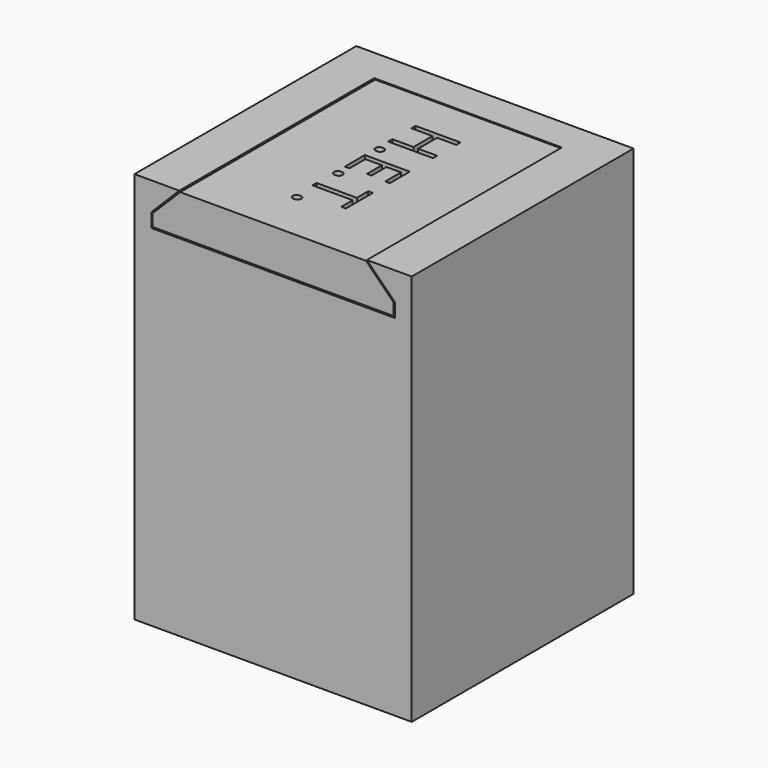
from build123d import *

# Parameters (mm, degrees)
F1_DEPTH      = 25
F2_W          = 19.8
F2_H          = 19.8
F3_DEPTH      = 1
F5_DEPTH      = 2
F7_DEPTH      = 1
F8_DEPTH      = 19.8
F10_DEPTH     = 2.4
F11_DEPTH     = 2
F13_DEPTH     = 17.4
F14_TEXT_SIZE = 4.4975727279
F15_DEPTH     = 3


# Not quite as in the source:
# - Text() gives the source's letters only with a copy of the font that has no kerning and outlines rounded to 1/6400 em; it was checked with that copy


with BuildPart() as f1:
    # F0 (on Top) → F1 (new body)
    with BuildSketch(Plane.XY):
        Polygon((0, -7.5), (-7.5, -7.5), (-7.5, 0), (-7.5, 7.5), (-7.5, 9.9), (-9.9, 9.9), (-9.9, -9.9), (9.9, -9.9), (9.9, -7.5), (7.5, -7.5), align=None)
        Polygon((7.5, 7.5), (7.5, -7.5), (9.9, -7.5), (9.9, 9.9), (-7.5, 9.9), (-7.5, 7.5), align=None)
    extrude(amount=F1_DEPTH)

    # F2 (on face) → F3 (join)
    with BuildSketch(Plane(origin=(0, 0, 0), x_dir=(1, 0, 0), z_dir=(0, 0, -1))):
        Rectangle(F2_W, F2_H)
    extrude(amount=F3_DEPTH)

    # F4 (on face) → F5 (cut)
    with BuildSketch(Plane.XY.offset(25)):
        Polygon((-8.7, 7.5), (-8.7, 0), (-8.7, -9.9), (8.7, -9.9), (8.7, 0), (8.7, 7.5), (7.5, 7.5), (7.5, -7.5), (-7.5, -7.5), (-7.5, 7.5), align=None)
    extrude(amount=-F5_DEPTH, mode=Mode.SUBTRACT)

    # F7 (add): a face of the model
    f7_faces = [f1.faces().sort_by_distance(p)[0] for p in [
        (-8.4539268401, -1.2, 23),
    ]]
    extrude(f7_faces, amount=F7_DEPTH)

    # F6 (on face) → F8 (join, through all)
    with BuildSketch(Plane.XZ.offset(9.9)):
        Polygon((-9.9, 27), (-9.9, 25), (-8.7, 25), (-6.7, 27), align=None)
        Polygon((9.9, 27), (6.7, 27), (8.7, 25), (9.9, 25), align=None)
    extrude(amount=-F8_DEPTH)

    # F9 (on face) → F10 (join, through all)
    with BuildSketch(Plane(origin=(0, 9.9, 0), x_dir=(-1, 0, 0), z_dir=(0, 1, 0))):
        Polygon((-6.7, 25), (-6.7, 27), (-8.7, 25), align=None)
        Polygon((6.7, 27), (6.7, 25), (8.7, 25), align=None)
    extrude(amount=-F10_DEPTH)

    # F11 (add, through all): a face of the model
    f11_faces = [f1.faces().sort_by_distance(p)[0] for p in [
        (0, 8.7, 25),
    ]]
    extrude(f11_faces, amount=F11_DEPTH)


with BuildPart() as f13:
    # F12 (on face) → F13 (new body, through all)
    with BuildSketch(Plane.XZ.offset(9.9)):
        Polygon((-8.6, 24.9585786438), (-8.6, 24.1), (8.6, 24.1), (8.6, 24.9585786438), (6.6292893219, 26.9292893219), (-6.6292893219, 26.9292893219), align=None)
    extrude(amount=-F13_DEPTH)

    # F14 (on face) → F15 (cut)
    with BuildSketch(Plane.XY.offset(26.9292893219)):
        with Locations(Location((-1.3924839441, 4.9880119721), (0, 0, -90))):
            Text('H.E.T.', F14_TEXT_SIZE, font='Open Sans', text_align=(TextAlign.LEFT, TextAlign.BOTTOM))
    extrude(amount=-F15_DEPTH, mode=Mode.SUBTRACT)


solid = Compound([f1.part, f13.part])
